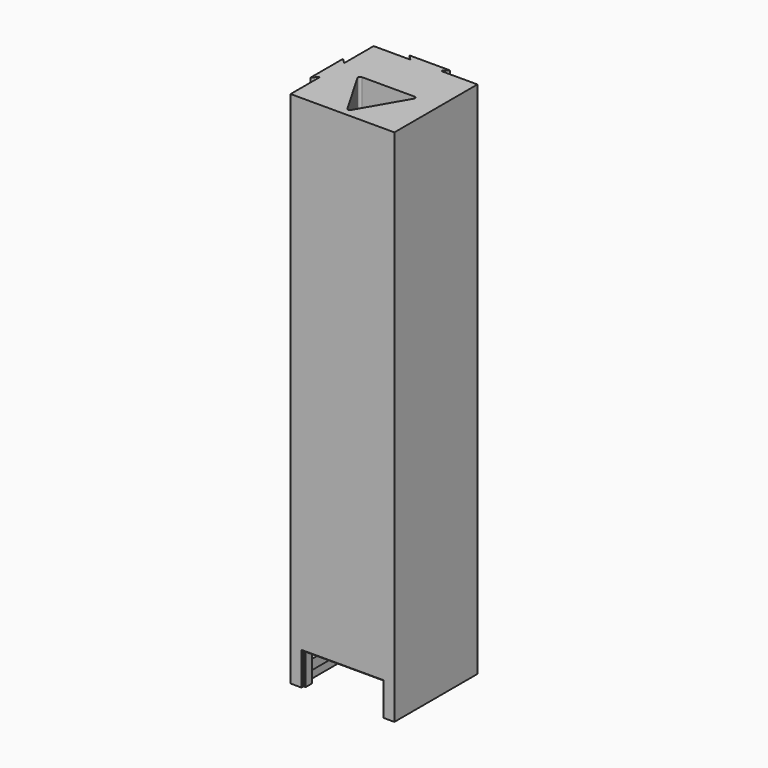
from build123d import *

# Parameters (mm, degrees)
F1_DEPTH = 127
F3_DEPTH = 7.62
F5_DEPTH = 0.635
F6_W     = 20.32
F6_H     = 2.413
F7_DEPTH = 1.016


# Not quite as in the source:
# - a feature names something its author has since deleted; it is built from what else it names


with BuildPart() as f1:
    # F0 (on Top) → F1 (new body)
    with BuildSketch(Plane.XY):
        Polygon((12.7, -12.7), (12.7, 12.7), (3.683, 12.7), (-3.683, 12.7), (-12.7, 12.7), (-12.7, 3.683), (-12.7, -3.683), (-12.7, -12.7), align=None)
        with BuildLine():
            ThreePointArc((-6.8924075136, 0.508), (-6.8924075136, 1.016), (-6.4524666085, 1.27))
            Line((-6.4524666085, 1.27), (6.4524666085, 1.27))
            ThreePointArc((6.4524666085, 1.27), (6.8924075136, 1.016), (6.8924075136, 0.508))
            Line((6.8924075136, 0.508), (0.4399409051, -10.668))
            ThreePointArc((0.4399409051, -10.668), (0, -10.922), (-0.4399409051, -10.668))
            Line((-0.4399409051, -10.668), (-6.8924075136, 0.508))
        make_face(mode=Mode.SUBTRACT)
        Polygon((-13.97, -4.953), (-12.7, -3.683), (-12.7, 3.683), (-13.97, 4.953), align=None)
        Polygon((-3.683, 12.7), (3.683, 12.7), (4.953, 13.97), (-4.953, 13.97), align=None)
    extrude(amount=F1_DEPTH)

    # F2 (on face) → F3 (cut)
    with BuildSketch(Plane(origin=(0, 0, 0), x_dir=(1, 0, 0), z_dir=(0, 0, -1))):
        Polygon((9.525, 12.7), (-9.525, 12.7), (-9.525, 10.16), (-10.795, 10.16), (-10.795, -10.16), (10.795, -10.16), (10.795, 10.16), (9.525, 10.16), align=None)
        with BuildLine():
            ThreePointArc((-6.4524666085, -1.27), (-6.8924075136, -1.016), (-6.8924075136, -0.508))
            Line((-6.8924075136, -0.508), (-0.4399409051, 10.668))
            ThreePointArc((-0.4399409051, 10.668), (0, 10.922), (0.4399409051, 10.668))
            Line((0.4399409051, 10.668), (6.8924075136, -0.508))
            ThreePointArc((6.8924075136, -0.508), (6.8924075136, -1.016), (6.4524666085, -1.27))
            Line((6.4524666085, -1.27), (-6.4524666085, -1.27))
        make_face(mode=Mode.SUBTRACT)
    extrude(amount=-F3_DEPTH, mode=Mode.SUBTRACT)

    # F4 (on face) → F5 (cut)
    with BuildSketch(Plane.XZ.offset(12.7)):
        Polygon((10.033, 8.128), (-10.033, 8.128), (-10.033, 0), (-9.525, 0), (-9.525, 7.62), (9.525, 7.62), (9.525, 0), (10.033, 0), align=None)
    extrude(amount=-F5_DEPTH, mode=Mode.SUBTRACT)



with BuildPart() as f7:
    # F6 (on face) → F7 (new body)
    with BuildSketch(Plane.YZ.offset(-10.795)):
        with Locations((0, 3.8735)):
            Rectangle(F6_W, F6_H)
    extrude(amount=F7_DEPTH)


with BuildPart() as f1_1:
    add(f1.part)

    add(f7.part)  # F8 merges F7
    # F8: F7 across plane
    add(f7.part.mirror(Plane.YZ))


with BuildPart() as f9_1:
    # F9: copy of F1
    add(f1_1.part)


solid = f1_1.part
